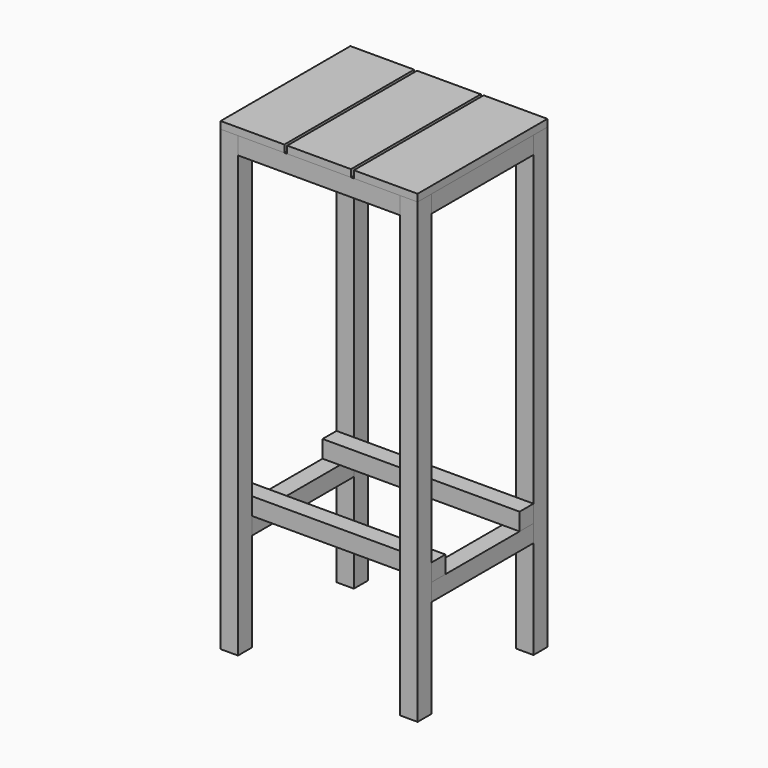
from build123d import *

# Parameters (mm, degrees)
F0_W      = 38.1
F0_H      = 38.1
F1_DEPTH  = 1003.3
F2_W      = 38.1
F2_H      = 38.1
F3_DEPTH  = 15.875
F4_W      = 355.6
F4_H      = 38.1
F5_DEPTH  = 38.1
F4_W_2    = 38.1
F4_H_2    = 279.4
F7_W      = 38.1
F7_H      = 203.2
F7_H_2    = 38.1
F8_DEPTH  = 38.1
F7_W_2    = 355.6
F9_DEPTH  = 38.1
F10_W     = 6.35
F10_H     = 355.6
F11_DEPTH = 1019.176


with BuildPart() as f1:
    # F0 (on Top) → F1 (new body)
    with BuildSketch(Plane.XY):
        with Locations((-196.85, 158.75)):
            Rectangle(F0_W, F0_H)
    extrude(amount=F1_DEPTH)


with BuildPart() as f1b:
    # F0 (on Top) → F1, piece 2 (new body)
    with BuildSketch(Plane.XY):
        with Locations((-196.85, -158.75)):
            Rectangle(F0_W, F0_H)
    extrude(amount=F1_DEPTH)


with BuildPart() as f1c:
    # F0 (on Top) → F1, piece 3 (new body)
    with BuildSketch(Plane.XY):
        with Locations((196.85, -158.75)):
            Rectangle(F0_W, F0_H)
    extrude(amount=F1_DEPTH)


with BuildPart() as f1d:
    # F0 (on Top) → F1, piece 4 (new body)
    with BuildSketch(Plane.XY):
        with Locations((196.85, 158.75)):
            Rectangle(F0_W, F0_H)
    extrude(amount=F1_DEPTH)


with BuildPart() as f3:
    # F2 (on face) → F3 (new body)
    with BuildSketch(Plane.XY.offset(1003.3)):
        Polygon((215.9, -177.8), (215.9, 177.8), (-215.9, 177.8), (-215.9, -139.7), (-177.8, -139.7), (-177.8, -177.8), align=None)
        with Locations((-196.85, -158.75)):
            Rectangle(F2_W, F2_H)
    extrude(amount=F3_DEPTH)

    # F10 (on face) → F11 (cut, through all)
    with BuildSketch(Plane.XY.offset(1019.175)):
        with Locations((-73.025, 0)):
            Rectangle(F10_W, F10_H)
        with Locations((73.025, 0)):
            Rectangle(F10_W, F10_H)
    extrude(amount=-F11_DEPTH, mode=Mode.SUBTRACT)


with BuildPart() as f5:
    # F4 (on face) → F5 (new body)
    with BuildSketch(Plane(origin=(0, 0, 1003.3), x_dir=(1, 0, 0), z_dir=(0, 0, -1))):
        with Locations((0, 158.75)):
            Rectangle(F4_W, F4_H)
    extrude(amount=F5_DEPTH)


with BuildPart() as f5b:
    # F4 (on face) → F5, piece 2 (new body)
    with BuildSketch(Plane(origin=(0, 0, 1003.3), x_dir=(1, 0, 0), z_dir=(0, 0, -1))):
        with Locations((0, -158.75)):
            Rectangle(F4_W, F4_H)
    extrude(amount=F5_DEPTH)


with BuildPart() as f5c:
    # F4 (on face) → F5, piece 3 (new body)
    with BuildSketch(Plane(origin=(0, 0, 1003.3), x_dir=(1, 0, 0), z_dir=(0, 0, -1))):
        with Locations((-196.85, 0)):
            Rectangle(F4_W_2, F4_H_2)
    extrude(amount=F5_DEPTH)


with BuildPart() as f5d:
    # F4 (on face) → F5, piece 4 (new body)
    with BuildSketch(Plane(origin=(0, 0, 1003.3), x_dir=(1, 0, 0), z_dir=(0, 0, -1))):
        with Locations((196.85, 0)):
            Rectangle(F4_W_2, F4_H_2)
    extrude(amount=F5_DEPTH)


with BuildPart() as f8:
    # F7 (on offset) → F8 (new body)
    with BuildSketch(Plane(origin=(0, 0, 254), x_dir=(1, 0, 0), z_dir=(0, 0, -1))):
        with Locations((196.85, 0)):
            Rectangle(F7_W, F7_H)
        with Locations((196.85, -120.65)):
            Rectangle(F7_W, F7_H_2)
        with Locations((196.85, 120.65)):
            Rectangle(F7_W, F7_H_2)
    extrude(amount=F8_DEPTH)


with BuildPart() as f8b:
    # F7 (on offset) → F8, piece 2 (new body)
    with BuildSketch(Plane(origin=(0, 0, 254), x_dir=(1, 0, 0), z_dir=(0, 0, -1))):
        with Locations((-196.85, 120.65)):
            Rectangle(F7_W, F7_H_2)
        with Locations((-196.85, 0)):
            Rectangle(F7_W, F7_H)
        with Locations((-196.85, -120.65)):
            Rectangle(F7_W, F7_H_2)
    extrude(amount=F8_DEPTH)


with BuildPart() as f9:
    # F7 (on offset) → F9 (new body)
    with BuildSketch(Plane(origin=(0, 0, 254), x_dir=(1, 0, 0), z_dir=(0, 0, -1))):
        with Locations((196.85, 120.65)):
            Rectangle(F7_W, F7_H_2)
        with Locations((0, 120.65)):
            Rectangle(F7_W_2, F7_H_2)
        with Locations((-196.85, 120.65)):
            Rectangle(F7_W, F7_H_2)
    extrude(amount=-F9_DEPTH)


with BuildPart() as f9b:
    # F7 (on offset) → F9, piece 2 (new body)
    with BuildSketch(Plane(origin=(0, 0, 254), x_dir=(1, 0, 0), z_dir=(0, 0, -1))):
        with Locations((-196.85, -120.65)):
            Rectangle(F7_W, F7_H_2)
        with Locations((0, -120.65)):
            Rectangle(F7_W_2, F7_H_2)
        with Locations((196.85, -120.65)):
            Rectangle(F7_W, F7_H_2)
    extrude(amount=-F9_DEPTH)


solid = Compound([f1.part, f1b.part, f1c.part, f1d.part, f3.part, f5.part, f5b.part, f5c.part, f5d.part, f8.part, f8b.part, f9.part, f9b.part])
